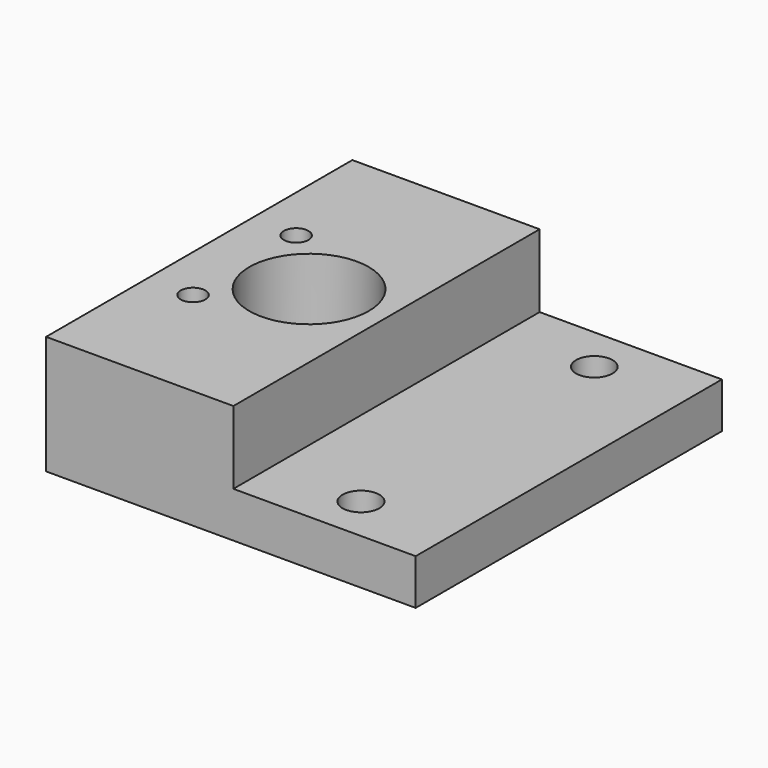
from build123d import *

# Parameters (mm, degrees)
F0_W     = 20
F0_H     = 42
F0_R     = 2.0193883272
F0_R_2   = 2
F1_DEPTH = 5
F0_W_2   = 20.55
F0_R_3   = 1.35
F0_R_4   = 6.55
F2_DEPTH = 13


# Not quite as in the source:
# - a feature of the source that left no trace in its solid (it failed there, or was rolled back) is left out


with BuildPart() as f1:
    # F0 (on Top) → F1 (new body)
    with BuildSketch(Plane.XY):
        with Locations((13.4585087977, 14.1658929903)):
            Rectangle(F0_W, F0_H)
        with Locations((13.4585087977, -1.8341070097)):
            Circle(F0_R, mode=Mode.SUBTRACT)
        with Locations((13.4585087977, 30.1658929903)):
            Circle(F0_R_2, mode=Mode.SUBTRACT)
    extrude(amount=F1_DEPTH)

    # F0 (on Top) → F2 (join)
    with BuildSketch(Plane.XY):
        with Locations((-6.8164912023, 14.1658929903)):
            Rectangle(F0_W_2, F0_H)
        with Locations((-12.1125590142, 7.0948251784)):
            Circle(F0_R_3, mode=Mode.SUBTRACT)
        with Locations((-5.0414912023, 14.1658929903)):
            Circle(F0_R_4, mode=Mode.SUBTRACT)
        with Locations((-12.1125590142, 21.2369608022)):
            Circle(F0_R_3, mode=Mode.SUBTRACT)
    extrude(amount=F2_DEPTH)


solid = f1.part
